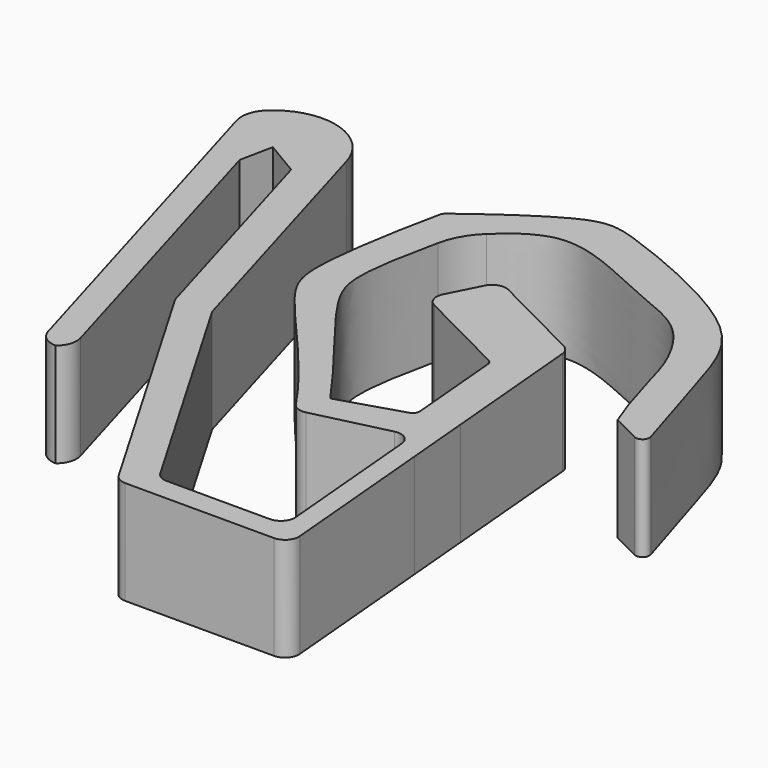
from build123d import *

# Parameters (mm, degrees)
F1_DEPTH    = 7.5
F2_T1_DEPTH = 15.2889844522
F2_T3_DEPTH = 14.7217373581
F3_R        = 5
F4_R        = 2


# Not quite as in the source:
# - a fillet or chamfer that OpenCascade refuses, or shapes differently, is made with other operations: its cross-section is extruded or revolved along the edge and cut away or added
# - the dataset's text gives a spline's control points without its knots; the knots are read off the source's solid


with BuildPart() as f1:
    # F0 (on Top) → F1 (new body)
    with BuildSketch(Plane.XY):
        with BuildLine():
            Line((-30.4297231978, 37.2361281484), (-27.9068994648, 35.7413323143))
            Line((-27.9068994648, 35.7413323143), (-23.1022062055, 19.2465248053))
            Line((-23.1022062055, 19.2465248053), (-12.1421488415, 0.4418746424))
            ThreePointArc((-12.1421488415, 0.4418746424), (-11.7764047105, 0.0783760722), (-11.2781835948, -0.0545739178))
            Line((-11.2781835948, -0.0545739178), (-0.5164044179, -0.0545739178))
            ThreePointArc((-0.5164044179, -0.0545739178), (0.2211832141, 0.2701746585), (0.4797097793, 1.0334971119))
            Line((0.4797097793, 1.0334971119), (-0.5501098771, 12.6811181757))
            Line((-0.5501098771, 12.6811181757), (-0.9665210168, 17.3908740359))
            Line((-0.9665210168, 17.3908740359), (-1.8790748935, 27.7121780525))
            ThreePointArc((-1.8790748935, 27.7121780525), (-2.0470497932, 28.1846293722), (-2.4232402919, 28.5161509026))
            Line((-2.4232402919, 28.5161509026), (-9.1651293115, 31.931889425))
            ThreePointArc((-9.1651293115, 31.931889425), (-9.9282723264, 31.9901918821), (-10.50912199, 31.4917943441))
            Line((-10.50912199, 31.4917943441), (-11.6780597733, 29.1845776897))
            ThreePointArc((-11.6780597733, 29.1845776897), (-11.7363622304, 28.4214346748), (-11.2379646923, 27.8405850112))
            Line((-11.2379646923, 27.8405850112), (-4.6428148812, 24.499191048))
            ThreePointArc((-4.6428148812, 24.499191048), (-4.4547196319, 24.3334302828), (-4.370732182, 24.097204623))
            Line((-4.370732182, 24.097204623), (-3.7807636833, 17.4244542335))
            Line((-3.7807636833, 17.4244542335), (-3.7619000234, 17.2110996318))
            ThreePointArc((-3.7619000234, 17.2110996318), (-3.8447935162, 16.8884260354), (-4.1120023476, 16.6894561347))
            Line((-4.1120023476, 16.6894561347), (-8.7035508168, 15.2670730452))
            add(Edge.make_bspline(
                [(-15.5142657673, 35.3507988058), (-16.1010755157, 32.5985703523), (-17.1494817729, 28.0372519615), (-15.947461142, 24.3954661972), (-11.3028420672, 19.0091491745), (-8.7035508168, 15.2670730452)],
                knots=[0, 0, 0, 0, 0.3392145091, 0.5718363816, 1, 1, 1, 1], degree=3))
            add(Edge.make_bspline(
                [(-15.5142657673, 35.3507988058), (-15.0440821248, 35.8322924551), (-14.1012745944, 36.7950332484), (-12.8603615018, 37.7878852095), (-11.798829502, 38.3315249945), (-10.960746448, 38.5863831942), (-10.0673858916, 38.6529058616), (-9.1141266995, 38.5405856329), (-8.1216983172, 38.2884636716), (-7.1063789778, 37.9305416741), (-6.0852486156, 37.5030969594), (-5.0746543782, 37.0427025856), (-4.0904435755, 36.5841639606), (-3.1487348398, 36.1695070149), (-2.2640452318, 35.8087630666), (-1.4362912989, 35.4682005173), (-0.667516675, 35.1230266013), (0.0411482358, 34.745905475), (0.6890718757, 34.31218751), (1.2766173569, 33.7895061105), (1.8074190243, 33.1765478565), (2.2779053445, 32.5103349131), (2.6859571098, 31.8206108547), (3.0297312381, 31.1384148993), (3.3064025308, 30.4975143414), (3.5178737246, 29.9196286172), (3.6959800621, 29.3465425456), (3.8692027201, 28.7283066119), (4.0337210144, 28.1331983491), (4.1916693597, 27.5848116783), (4.3725168618, 26.9787861335), (4.6299932224, 26.1462091657), (4.8417441396, 25.4774887899), (4.9422006393, 25.1616837102)],
                knots=[0, 0, 0, 0, 0.0498708284, 0.0997416568, 0.1246770709, 0.1496124851, 0.1745478993, 0.1994833135, 0.2244187277, 0.2493541419, 0.2742895561, 0.2992249703, 0.3241603844, 0.3490957986, 0.3740312128, 0.398966627, 0.4239020412, 0.4488374554, 0.4737728696, 0.4987082838, 0.5236436979, 0.5485791121, 0.5735145263, 0.5984499405, 0.6233853547, 0.6483207689, 0.6732561831, 0.6981915973, 0.7231270114, 0.7355947185, 0.7480624256, 0.7729978398, 0.797933254, 0.797933254, 0.797933254, 0.797933254], degree=3))
            Line((4.9422006393, 25.1616837102), (5.6051399225, 23.3596070707))
            Line((5.6051399225, 23.3596070707), (7.6567647722, 22.3201633759))
            ThreePointArc((7.6567647722, 22.3201633759), (8.2052790129, 22.3841276621), (8.3603471538, 22.9141400901))
            Line((8.3603471538, 22.9141400901), (8.3424245162, 22.9719955723))
            add(Edge.make_bspline(
                [(8.3424245162, 22.9719955723), (7.7488944153, 24.8545905089), (6.67729679, 28.253534975), (5.6930167186, 31.8382348733), (3.5011406257, 36.8403453764), (-7.5398608959, 41.4475683268), (-10.9611276957, 42.1663875514), (-17.0110458735, 37.5497083277), (-17.7048493275, 37.0005035791)],
                knots=[0, 0, 0, 0, 0.0984429904, 0.1773696293, 0.2725166361, 0.412807835, 0.4962393226, 0.6112830896, 0.6112830896, 0.6112830896, 0.6112830896], degree=3))
            add(Edge.make_bspline(
                [(-17.7048493275, 37.0005035791), (-17.7345511384, 36.9769920565), (-17.7590976226, 36.9573783291), (-17.7796839194, 36.9397418581)],
                knots=[0.6112830896, 0.6112830896, 0.6112830896, 0.6112830896, 0.6162081274, 0.6162081274, 0.6162081274, 0.6162081274], degree=3))
            ThreePointArc((-17.7796839194, 36.9397418581), (-17.850702418, 36.8517272472), (-17.9001241505, 36.750003645))
            add(Edge.make_bspline(
                [(-17.9001241505, 36.750003645), (-17.907153429, 36.7248909598), (-17.9143126936, 36.695697636), (-17.9225929782, 36.6608311238)],
                knots=[0.6331345136, 0.6331345136, 0.6331345136, 0.6331345136, 0.6377615142, 0.6377615142, 0.6377615142, 0.6377615142], degree=3))
            add(Edge.make_bspline(
                [(-17.9225929782, 36.6608311238), (-18.145074403, 35.7240093049), (-19.9037327351, 27.1462156298), (-18.3649930119, 23.476055144), (-12.5997298189, 17.7007658301), (-9.8035750323, 13.5473699634)],
                knots=[0.6377615142, 0.6377615142, 0.6377615142, 0.6377615142, 0.7620835298, 0.8496665033, 1, 1, 1, 1], degree=3))
            ThreePointArc((-9.8035750323, 13.5473699634), (-9.3318550602, 13.126966392), (-8.7022699851, 13.0732865238))
            Line((-8.7022699851, 13.0732865238), (-3.3345946353, 14.3662985288))
            ThreePointArc((-3.3345946353, 14.3662985288), (-2.5168389495, 14.2061733755), (-2.1042906941, 13.4821786494))
            Line((-2.1042906941, 13.4821786494), (-1.1510458373, 2.7006453938))
            ThreePointArc((-1.1510458373, 2.7006453938), (-1.4095724025, 1.9373229405), (-2.1471600344, 1.6125743641))
            Line((-2.1471600344, 1.6125743641), (-9.6046174943, 1.6125743641))
            ThreePointArc((-9.6046174943, 1.6125743641), (-10.1028386099, 1.7455243541), (-10.468582741, 2.1090229244))
            Line((-10.468582741, 2.1090229244), (-20.5396115367, 19.3883278582))
            Line((-20.5396115367, 19.3883278582), (-26.1053241383, 38.4957615815))
            ThreePointArc((-26.1053241383, 38.4957615815), (-29.9052669683, 41.7096110505), (-34.3455150255, 39.4618141043))
            Line((-34.3455150255, 39.4618141043), (-25.8251781299, 10.2109734327))
            Line((-25.8251781299, 10.2109734327), (-24.8756555892, 10.5269434158))
            Line((-24.8756555892, 10.5269434158), (-23.9261330484, 10.8429133989))
            Line((-23.9261330484, 10.8429133989), (-30.9189620372, 34.8497254653))
            Line((-30.9189620372, 34.8497254653), (-30.4297231978, 37.2361281484))
        make_face()
    extrude(amount=F1_DEPTH)

    # F2: fillet of radius 1.5 on 2 edges, made by hand

    # F2_s2 → F2_t1 (cut)
    with BuildSketch(Plane.XY.offset(-3.8944922261)):
        with BuildLine():
            ThreePointArc((-24.3470714005, 10.7028389106), (-25.5174199076, 10.7977363038), (-26.2608354224, 11.7066117163))
            Line((-26.2608354224, 11.7066117163), (-25.8251781299, 10.2109734327))
            Line((-25.8251781299, 10.2109734327), (-24.3470714005, 10.7028389106))
        make_face()
    extrude(amount=F2_T1_DEPTH, mode=Mode.SUBTRACT)

    # F2_s4 → F2_t3 (cut)
    with BuildSketch(Plane.XY.offset(-3.6108686791)):
        with BuildLine():
            ThreePointArc((-24.3300627987, 12.2296290784), (-24.4418412958, 11.1134033384), (-25.2965939413, 10.3868689275))
            Line((-25.2965939413, 10.3868689275), (-23.9261330484, 10.8429133989))
            Line((-23.9261330484, 10.8429133989), (-24.3300627987, 12.2296290784))
        make_face()
    extrude(amount=F2_T3_DEPTH, mode=Mode.SUBTRACT)

    # F3
    f3_edges = [f1.edges().sort_by_distance(p)[0] for p in [
        (-15.514266, 35.350799, 3.75),
    ]]
    fillet(f3_edges, radius=F3_R)

    # F4
    f4_edges = [f1.edges().sort_by_distance(p)[0] for p in [
        (-34.345515, 39.461814, 3.75),
    ]]
    fillet(f4_edges, radius=F4_R)


solid = f1.part
